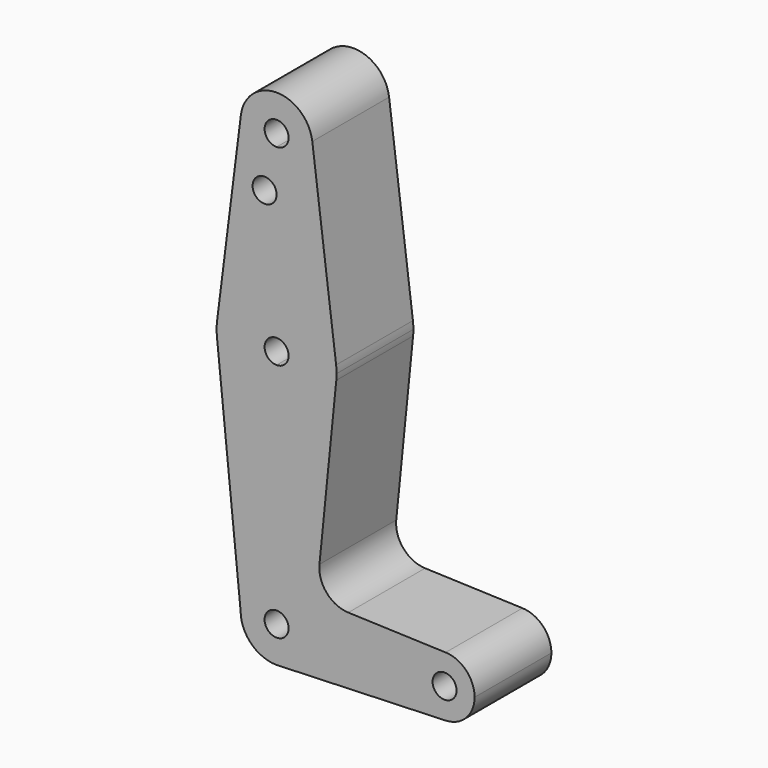
from build123d import *

# Parameters (mm, degrees)
F0_R     = 3.175
F1_DEPTH = 25.4


with BuildPart() as f1:
    # F0 (on Front) → F1 (new body)
    with BuildSketch(Plane.XZ):
        with BuildLine():
            Line((0.6773435479, -9.500885786), (0, -9.525))
            ThreePointArc((0, -9.525), (0.3388863295, -9.5189695375), (0.6773435479, -9.500885786))
        make_face()
        with BuildLine():
            Line((-15.7942028036, 61.9003804205), (-9.525, 0))
            ThreePointArc((-9.525, 0), (-6.7351920908, 6.7351920908), (0, 9.525))
            Line((0, 9.525), (0, 47.625))
            ThreePointArc((0, 47.625), (-10.644756084, 51.722700101), (-15.7942028036, 61.9003804205))
        make_face()
        with BuildLine():
            ThreePointArc((9.525, 0), (6.9705567315, -6.4912990883), (0.6773435479, -9.500885786))
            Line((0.6773435479, -9.500885786), (44.7324052746, -7.9324746146))
            ThreePointArc((44.7324052746, -7.9324746146), (38.9380895153, -5.7116327839), (36.5125, 0))
            Line((36.5125, 0), (9.525, 0))
        make_face()
        with BuildLine():
            Line((0, 100.0252), (0, 79.375))
            ThreePointArc((0, 79.375), (10.5003255158, 75.40625), (15.7504882737, 65.484375))
            Line((15.7504882737, 65.484375), (9.4502929642, 115.490625))
            ThreePointArc((9.4502929642, 115.490625), (9.5063048942, 114.896483242), (9.525, 114.3))
            ThreePointArc((9.525, 114.3), (6.7351920908, 107.5648079092), (0, 104.775))
            Line((0, 104.775), (0, 100.0252))
        make_face()
        with BuildLine():
            ThreePointArc((36.5125, 0), (38.9380895153, -5.7116327839), (44.7324052746, -7.9324746146))
            ThreePointArc((44.7324052746, -7.9324746146), (50.1616327839, -5.5119104847), (52.3875, 0))
            ThreePointArc((52.3875, 0), (50.1616327839, 5.5119104847), (44.7324052746, 7.9324746146))
            ThreePointArc((44.7324052746, 7.9324746146), (38.9380895153, 5.7116327839), (36.5125, 0))
        make_face()
        with BuildLine():
            ThreePointArc((47.625, 0), (44.45, -3.175), (41.275, 0))
            ThreePointArc((41.275, 0), (44.45, 3.175), (47.625, 0))
        make_face(mode=Mode.SUBTRACT)
        with BuildLine():
            ThreePointArc((9.4502929642, 115.490625), (0, 123.825), (-9.4502929642, 115.490625))
            ThreePointArc((-9.4502929642, 115.490625), (-7.14375, 107.9998046905), (0, 104.775))
            ThreePointArc((0, 104.775), (6.7351920908, 107.5648079092), (9.525, 114.3))
            ThreePointArc((9.525, 114.3), (9.5063048942, 114.896483242), (9.4502929642, 115.490625))
        make_face()
        with BuildLine():
            ThreePointArc((3.175, 114.3), (2.2450640303, 112.0549359697), (0, 111.125))
            ThreePointArc((0, 111.125), (-2.2450640303, 116.5450640303), (3.175, 114.3))
        make_face(mode=Mode.SUBTRACT)
        with BuildLine():
            Line((0, 60.325), (0, 47.625))
            ThreePointArc((0, 47.625), (10.6492737428, 51.7267849017), (15.7954255641, 61.9125))
            ThreePointArc((15.7954255641, 61.9125), (15.8550939106, 62.7052534459), (15.875, 63.5))
            ThreePointArc((15.875, 63.5), (15.8438414904, 64.4941387366), (15.7504882737, 65.484375))
            ThreePointArc((15.7504882737, 65.484375), (10.5003255158, 75.40625), (0, 79.375))
            Line((0, 79.375), (0, 66.675))
            ThreePointArc((0, 66.675), (2.2450640303, 65.7450640303), (3.175, 63.5))
            ThreePointArc((3.175, 63.5), (2.2450640303, 61.2549359697), (0, 60.325))
        make_face()
        with BuildLine():
            ThreePointArc((-15.7504882737, 65.484375), (-15.8738192656, 63.6936154008), (-15.7942028036, 61.9003804205))
            ThreePointArc((-15.7942028036, 61.9003804205), (-10.644756084, 51.722700101), (0, 47.625))
            Line((0, 47.625), (0, 60.325))
            ThreePointArc((0, 60.325), (-3.175, 63.5), (0, 66.675))
            Line((0, 66.675), (0, 79.375))
            ThreePointArc((0, 79.375), (-10.5003255158, 75.40625), (-15.7504882737, 65.484375))
        make_face()
        with BuildLine():
            Line((0, 47.625), (0, 9.525))
            ThreePointArc((0, 9.525), (6.7351920908, 6.7351920908), (9.525, 0))
            Line((9.525, 0), (36.5125, 0))
            ThreePointArc((36.5125, 0), (38.9380895153, 5.7116327839), (44.7324052746, 7.9324746146))
            Line((44.7324052746, 7.9324746146), (18.968327868, 8.8497055806))
            ThreePointArc((18.968327868, 8.8497055806), (13.2612039825, 11.5674628959), (11.3408358685, 17.5898921545))
            Line((11.3408358685, 17.5898921545), (15.7954255641, 61.9125))
            ThreePointArc((15.7954255641, 61.9125), (10.6492737428, 51.7267849017), (0, 47.625))
        make_face()
        with BuildLine():
            ThreePointArc((0, 9.525), (-6.7351920908, 6.7351920908), (-9.525, 0))
            ThreePointArc((-9.525, 0), (-6.7351920908, -6.7351920908), (0, -9.525))
            Line((0, -9.525), (0.6773435479, -9.500885786))
            ThreePointArc((0.6773435479, -9.500885786), (6.9705567315, -6.4912990883), (9.525, 0))
            Line((9.525, 0), (3.175, 0))
            ThreePointArc((3.175, 0), (-2.2450640303, -2.2450640303), (0, 3.175))
            Line((0, 3.175), (0, 9.525))
        make_face()
        with BuildLine():
            ThreePointArc((9.525, 0), (6.7351920908, 6.7351920908), (0, 9.525))
            Line((0, 9.525), (0, 3.175))
            ThreePointArc((0, 3.175), (2.2450640303, 2.2450640303), (3.175, 0))
            Line((3.175, 0), (9.525, 0))
        make_face()
        with BuildLine():
            Line((-9.4502929642, 115.490625), (-15.7504882737, 65.484375))
            ThreePointArc((-15.7504882737, 65.484375), (-10.5003255158, 75.40625), (0, 79.375))
            Line((0, 79.375), (0, 100.0252))
            Line((0, 100.0252), (0, 104.775))
            ThreePointArc((0, 104.775), (-7.14375, 107.9998046905), (-9.4502929642, 115.490625))
        make_face()
        with Locations((-3.175, 100.0252)):
            Circle(F0_R, mode=Mode.SUBTRACT)
    extrude(amount=F1_DEPTH)


solid = f1.part
